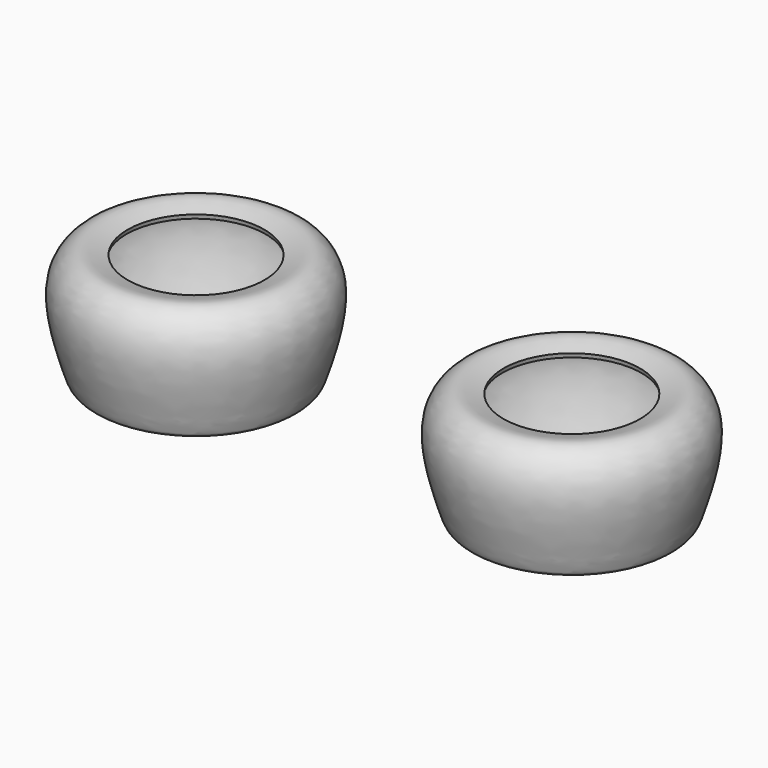
from build123d import *


# Not quite as in the source:
# - the dataset's text gives a spline's control points without its knots; the knots are read off the source's solid


with BuildPart() as f1:
    # F0 (on Front) → F1 (revolve)
    with BuildSketch(Plane.XZ):
        with BuildLine():
            add(Edge.make_bspline(
                [(0, 0), (-46.8283713472, 0), (-44.7840341326, -5.447146618), (-59.5277709578, 40.4415915376), (-44.5304306228, 56.1582427364), (-38.4018644691, 53.1126670539), (-31.8415872753, 51.3234995306)],
                knots=[0, 0, 0, 0, 0.3407554477, 0.6268715684, 0.8241882344, 1, 1, 1, 1], degree=3))
            Line((0, 0), (0, 2.099998523))
            add(Edge.make_bspline(
                [(0, 2.099998523), (-4.3026543874, 2.099998523), (-12.1009428415, 2.0500937671), (-21.6138081819, 1.8945496229), (-29.1753818063, 1.7274726147), (-35.0122882791, 1.6183219269), (-39.3371094254, 1.6348854777), (-41.8325043332, 1.8057342756), (-43.2259237668, 2.0422516271), (-43.9832849264, 2.2563395586), (-44.4836540739, 2.4830783318), (-44.8017721679, 2.7039497755), (-45.0516557494, 2.9564473297), (-45.3111982297, 3.3321191094), (-45.5933134285, 3.8992358776), (-45.8932874092, 4.6764355316), (-46.1635116134, 5.4953650392), (-46.4004315365, 6.2477745039), (-46.6565234083, 7.0665766189), (-47.0054362601, 8.1775924955), (-47.6119047951, 10.1266277263), (-48.4385730424, 12.8534614027), (-49.4663959956, 16.4857152405), (-50.455557884, 20.3692009201), (-51.3314837606, 24.3926822968), (-52.0201845889, 28.442112111), (-52.4493557531, 32.3998739667), (-52.5337184512, 35.5185789054), (-52.4078908487, 37.8415764594), (-52.2121228384, 39.47855828), (-51.9087103016, 41.0031554525), (-51.3692954928, 42.9142350629), (-50.4732808774, 45.0601390793), (-49.1320800619, 47.2391026366), (-47.6183554734, 49.0039830448), (-46.2973595732, 50.1133606739), (-45.263453908, 50.7755338661), (-44.5154286136, 51.159066835), (-43.8163038655, 51.4289329421), (-43.1717300914, 51.5948552885), (-42.5346627794, 51.6793942733), (-41.6369667721, 51.6947891058), (-40.3236990396, 51.5272452082), (-38.2865910168, 51.0136652528), (-35.7142066115, 50.2446759031), (-33.5822571176, 49.6215308456), (-32.3941337308, 49.2974970106)],
                knots=[0, 0, 0, 0, 0.03125, 0.0625, 0.09375, 0.125, 0.15625, 0.1875, 0.2031250001, 0.2187500001, 0.2343750001, 0.2500000001, 0.2656250001, 0.2812500001, 0.2968750001, 0.3125000001, 0.3281250001, 0.3359375001, 0.3437500001, 0.3593750001, 0.3750000001, 0.4062500001, 0.4375000001, 0.4687500001, 0.5000000001, 0.5312500001, 0.5625000001, 0.5937500001, 0.6093750002, 0.6250000002, 0.6406250002, 0.6562500002, 0.6875000002, 0.7187500002, 0.7500000002, 0.7812500002, 0.7968750002, 0.8125000002, 0.8281250002, 0.8437500002, 0.8593750002, 0.8750000002, 0.9062500002, 0.9375000002, 0.9687500002, 1.0000000003, 1.0000000003, 1.0000000003, 1.0000000003], degree=3))
            Line((-32.3941337308, 49.2974970106), (-31.8415872753, 51.3234995306))
        make_face()
    revolve(axis=Axis((0, 0, 1.0499992615), (0, 0, -1)))


with BuildPart() as f2_1:
    # F2: copy of F1
    add(f1.part.moved(Location((175, 0, 0))))


solid = Compound([f1.part, f2_1.part])
